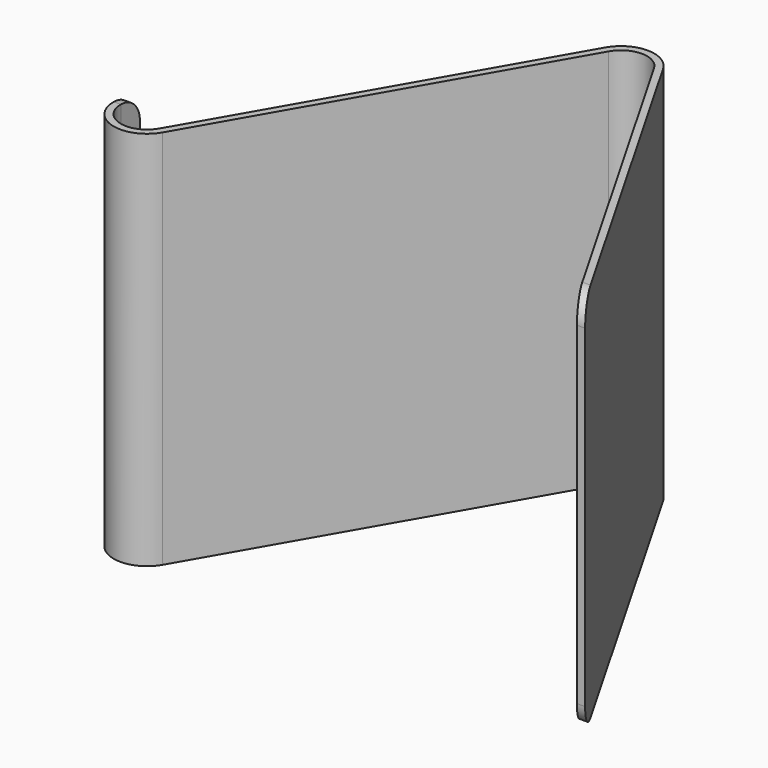
from build123d import *

# Parameters (mm, degrees)
F1_DEPTH    = 40
F2_T1_DEPTH = 14
F2_T3_DEPTH = 26.7295341336


# Not quite as in the source:
# - a fillet or chamfer that OpenCascade refuses, or shapes differently, is made with other operations: its cross-section is extruded or revolved along the edge and cut away or added


with BuildPart() as f1:
    # F0 (on Top) → F1 (new body, symmetric)
    with BuildSketch(Plane.XY):
        with BuildLine():
            Line((-7, 5), (-7, 0))
            ThreePointArc((-7, 0), (-1.8031925829, -6.7637634871), (6.0709990026, -3.484676615))
            Line((6.0709990026, -3.484676615), (45.2299293551, 64.7379601975))
            ThreePointArc((45.2299293551, 64.7379601975), (50, 67.5), (54.7700706449, 64.7379601975))
            Line((54.7700706449, 64.7379601975), (95.9467521433, -7))
            Line((95.9467521433, -7), (97.6762862769, -7))
            Line((97.6762862769, -7), (56.0709990026, 65.484676615))
            ThreePointArc((56.0709990026, 65.484676615), (50, 69), (43.9290009974, 65.484676615))
            Line((43.9290009974, 65.484676615), (4.7700706449, -2.7379601975))
            ThreePointArc((4.7700706449, -2.7379601975), (-1.4167941723, -5.314385597), (-5.5, 0))
            Line((-5.5, 0), (-5.5, 5))
            Line((-5.5, 5), (-7, 5))
        make_face()
    extrude(amount=F1_DEPTH, both=True)

    # F2: fillet of radius 5 on 4 edges, made by hand

    # F2_s2 → F2_t1 (cut)
    with BuildSketch(Plane.YZ.offset(-19.5)):
        with BuildLine():
            ThreePointArc((5, 35), (3.5355339059, 38.5355339059), (0, 40))
            Line((0, 40), (5, 40))
            Line((5, 40), (5, 35))
        make_face()
        with BuildLine():
            ThreePointArc((5, -35), (3.5355339059, -38.5355339059), (0, -40))
            Line((0, -40), (5, -40))
            Line((5, -40), (5, -35))
        make_face()
    extrude(amount=F2_T1_DEPTH, mode=Mode.SUBTRACT)

    # F2_s4 → F2_t3 (cut)
    with BuildSketch(Plane.YZ.offset(83.4467521433)):
        with BuildLine():
            ThreePointArc((-7, 35), (-5.5355339059, 38.5355339059), (-2, 40))
            Line((-2, 40), (-7, 40))
            Line((-7, 40), (-7, 35))
        make_face()
        with BuildLine():
            ThreePointArc((-7, -35), (-5.5355339059, -38.5355339059), (-2, -40))
            Line((-2, -40), (-7, -40))
            Line((-7, -40), (-7, -35))
        make_face()
    extrude(amount=F2_T3_DEPTH, mode=Mode.SUBTRACT)


solid = f1.part
